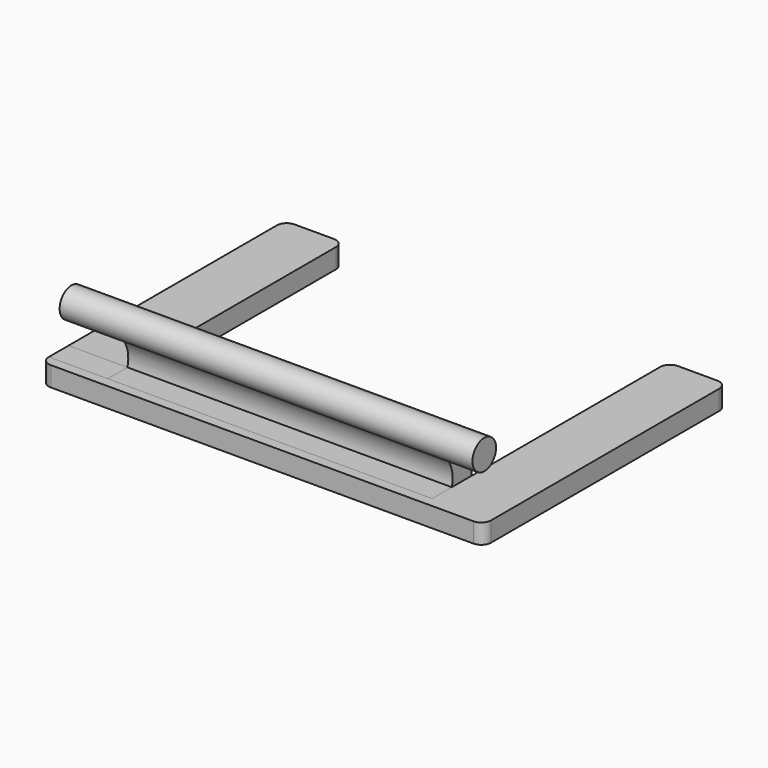
from build123d import *
from build123d import SkipClean  # not in build123d's __all__

# Parameters (mm, degrees)
F1_DEPTH    = 2
F2_W        = 33
F2_H        = 5
F3_DEPTH    = 5
F6_R        = 1.5
F7_DEPTH    = 42
F8_T1_DEPTH = 54.6506350946
F10_DEPTH   = 39.001


# Not quite as in the source:
# - a fillet or chamfer that OpenCascade refuses, or shapes differently, is made with other operations: its cross-section is extruded or revolved along the edge and cut away or added


with BuildPart() as f1:
    # F0 (on Top) → F1 (new body)
    with BuildSketch(Plane.XY):
        with BuildLine():
            Line((-21.5, -15.5), (21.5, -15.5))
            ThreePointArc((21.5, -15.5), (22.2071067812, -15.2071067812), (22.5, -14.5))
            Line((22.5, -14.5), (22.5, 14.5))
            ThreePointArc((22.5, 14.5), (22.2071067812, 15.2071067812), (21.5, 15.5))
            Line((21.5, 15.5), (17.5, 15.5))
            ThreePointArc((17.5, 15.5), (16.7928932188, 15.2071067812), (16.5, 14.5))
            Line((16.5, 14.5), (16.5, -9.5))
            Line((16.5, -9.5), (-16.5, -9.5))
            Line((-16.5, -9.5), (-16.5, 14.5))
            ThreePointArc((-16.5, 14.5), (-16.7928932188, 15.2071067812), (-17.5, 15.5))
            Line((-17.5, 15.5), (-21.5, 15.5))
            ThreePointArc((-21.5, 15.5), (-22.2071067812, 15.2071067812), (-22.5, 14.5))
            Line((-22.5, 14.5), (-22.5, -14.5))
            ThreePointArc((-22.5, -14.5), (-22.2071067812, -15.2071067812), (-21.5, -15.5))
        make_face()
    extrude(amount=F1_DEPTH)

    # F2 (on face) → F3 (join)
    with BuildSketch(Plane.XY.offset(2)):
        with Locations((0, -12)):
            Rectangle(F2_W, F2_H)
    extrude(amount=F3_DEPTH)

    # F6 (on offset) → F7 (join, through all)
    with BuildSketch(Plane.YZ.offset(21)):
        with Locations((-13.5, 7)):
            Circle(F6_R)
    extrude(amount=-F7_DEPTH)

    # F8: fillet of radius 5 on 1 edges, made by hand

    # F8_s2 → F8_t1 (cut)
    with BuildSketch(Plane.YZ.offset(-27.3253175473)):
        with BuildLine():
            ThreePointArc((-9.5, 2.6698729811), (-10.1698729811, 5.1698729811), (-12, 7))
            Line((-12, 7), (-9.5, 7))
            Line((-9.5, 7), (-9.5, 2.6698729811))
        make_face()
    extrude(amount=F8_T1_DEPTH, mode=Mode.SUBTRACT)

    # F9 (on face) → F10 (cut, through all)
    with BuildSketch(Plane.YZ.offset(16.5)):
        with BuildLine():
            ThreePointArc((-13.6298629558, 5.5056320357), (-14.0954446994, 5.6232481669), (-14.5, 5.8819660113))
            Line((-14.5, 5.8819660112), (-14.5, 2))
            Line((-14.5, 2), (-12, 2))
            ThreePointArc((-12, 2), (-12.1749548088, 4.0503584453), (-13.6298629558, 5.5056320357))
        make_face()
    with SkipClean():  # cleaning this boolean's faces spoils the solid; the shape is the same uncleaned
        extrude(amount=-F10_DEPTH, mode=Mode.SUBTRACT)


solid = f1.part
